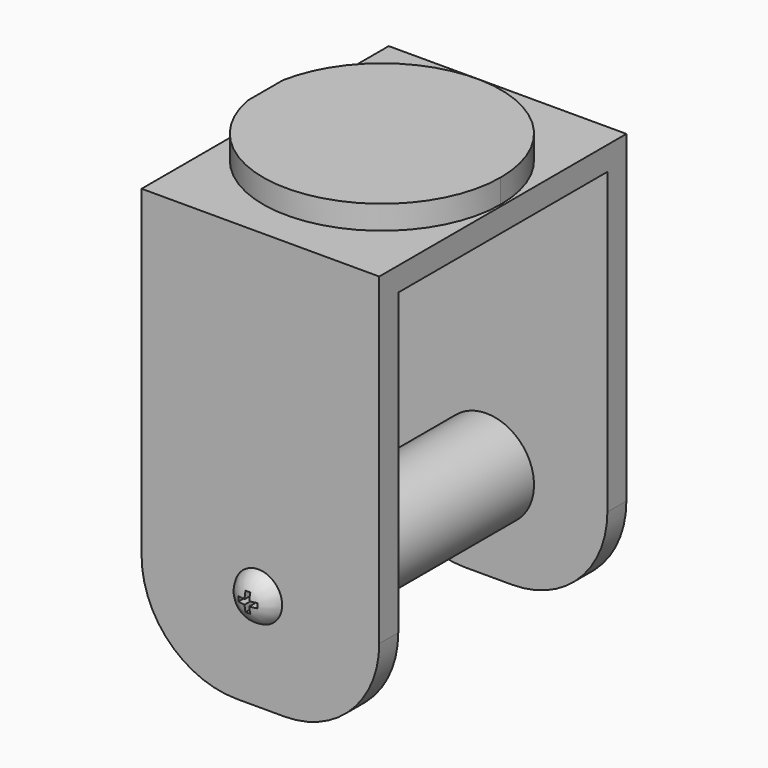
from build123d import *

# Parameters (mm, degrees)
F1_DEPTH  = 5
F2_W      = 50
F2_H      = 55
F2_H_2    = 5
F3_DEPTH  = 5
F7_DEPTH  = 5
F8_R      = 10
F9_DEPTH  = 55
F10_R     = 5
F11_DEPTH = 3
F12_W     = 1.5
F12_H     = 1
F12_W_2   = 1
F12_H_2   = 1.5
F14_DEPTH = 3
F15_R     = 5
F16_DEPTH = 3
F18_DEPTH = 3


# Not quite as in the source:
# - a fillet or chamfer that OpenCascade refuses, or shapes differently, is made with other operations: its cross-section is extruded or revolved along the edge and cut away or added


with BuildPart() as f1:
    # F0 (on Front) → F1 (new body)
    with BuildSketch(Plane.XZ):
        with BuildLine():
            Line((25.4373252392, 36.0385786295), (-24.5626747608, 36.0385786295))
            Line((-24.5626747608, 36.0385786295), (-24.5626747608, -26.9614213705))
            ThreePointArc((-24.5626747608, -26.9614213705), (-18.7048103845, -41.1035569942), (-4.5626747608, -46.9614213705))
            Line((-4.5626747608, -46.9614213705), (5.4373252392, -46.9614213705))
            ThreePointArc((5.4373252392, -46.9614213705), (19.5794608629, -41.1035569942), (25.4373252392, -26.9614213705))
            Line((25.4373252392, -26.9614213705), (25.4373252392, 36.0385786295))
        make_face()
    extrude(amount=F1_DEPTH)

    # F2 (on face) → F3 (join)
    with BuildSketch(Plane.XY.offset(36.0385786295)):
        with Locations((0.4373252392, 27.5)):
            Rectangle(F2_W, F2_H)
        with Locations((0.4373252392, -2.5)):
            Rectangle(F2_W, F2_H_2)
    extrude(amount=F3_DEPTH)

    # F5: F1 across plane


with BuildPart() as f1_1:
    add(f1.part)
    add(f1.part.mirror(Plane(origin=(0.4373252392, 27.5, -3.8633044256), x_dir=(1, 0, 0), z_dir=(0, 1, 0))))

    # F6 (on face) → F7 (join)
    with BuildSketch(Plane.XY.offset(41.0385786295)):
        with BuildLine():
            ThreePointArc((-24.5626747608, 22.8443573382), (2.3380687521, 2.6095714278), (25, 27.5))
            ThreePointArc((25, 27.5), (2.3380687521, 52.3904285722), (-24.5626747608, 32.1556426618))
            Line((-24.5626747608, 32.1556426618), (-24.5626747608, 22.8443573382))
        make_face()
    extrude(amount=F7_DEPTH)

    # F8 (on face) → F9 (join, through all)
    with BuildSketch(Plane(origin=(0, 0, 0), x_dir=(-1, 0, 0), z_dir=(0, 1, 0))):
        with Locations((0, -26.9662032763)):
            Circle(F8_R)
    extrude(amount=F9_DEPTH)

    # F10 (on face) → F11 (join)
    with BuildSketch(Plane.XZ.offset(5)):
        with Locations((0, -26.4660866176)):
            Circle(F10_R)
    extrude(amount=F11_DEPTH)

    # F13: fillet of radius 5 on 1 edges, made by hand

    # F13_s1 → F13_t2 (revolve, cut)
    with BuildSketch(Plane.XY.offset(-26.4660866176)):
        with BuildLine():
            ThreePointArc((5, -5), (3.1560370926, -7.1833001327), (0.417424305, -8))
            Line((0.417424305, -8), (5, -8))
            Line((5, -8), (5, -5))
        make_face()
    revolve(axis=Axis((0, -8, -26.4660866176), (0, -1, 0)), mode=Mode.SUBTRACT)

    # F12 (on face) → F14 (cut)
    with BuildSketch(Plane.XZ.offset(8)):
        with Locations((-1.25, -26.4660866176)):
            Rectangle(F12_W, F12_H)
        Polygon((1, -25.9660866176), (0.5, -25.9660866176), (0.5, -26.9660866176), (1, -26.9660866176), (2, -26.9660866176), (2, -25.9660866176), align=None)
        with Locations((0, -26.4660866176)):
            Rectangle(F12_W_2, F12_H)
        with Locations((0, -25.2160866176)):
            Rectangle(F12_W_2, F12_H_2)
        with Locations((0, -27.7160866176)):
            Rectangle(F12_W_2, F12_H_2)
    extrude(amount=-F14_DEPTH, mode=Mode.SUBTRACT)

    # F15 (on face) → F16 (join)
    with BuildSketch(Plane(origin=(0, 60, 0), x_dir=(-1, 0, 0), z_dir=(0, 1, 0))):
        with Locations((0, -26.4660866176)):
            Circle(F15_R)
    extrude(amount=F16_DEPTH)

    # F17 (on face) → F18 (cut)
    with BuildSketch(Plane(origin=(0, 63, 0), x_dir=(-1, 0, 0), z_dir=(0, 1, 0))):
        Polygon((0.5, -24.4660866176), (-0.5, -24.4660866176), (-0.5, -25.9660866176), (-2, -25.9660866176), (-2, -26.9660866176), (-0.5, -26.9660866176), (-0.5, -28.4660866176), (0.5, -28.4660866176), (0.5, -26.9660866176), (2, -26.9660866176), (2, -25.9660866176), (0.5, -25.9660866176), align=None)
    extrude(amount=-F18_DEPTH, mode=Mode.SUBTRACT)

    # F19: fillet of radius 5 on 1 edges, made by hand

    # F19_s1 → F19_t2 (revolve, cut)
    with BuildSketch(Plane.XY.offset(-26.4660866176)):
        with BuildLine():
            ThreePointArc((-5, 60), (-3.1560370926, 62.1833001327), (-0.417424305, 63))
            Line((-0.417424305, 63), (-5, 63))
            Line((-5, 63), (-5, 60))
        make_face()
    revolve(axis=Axis((0, 63, -26.4660866176), (0, 1, 0)), mode=Mode.SUBTRACT)


solid = f1_1.part
